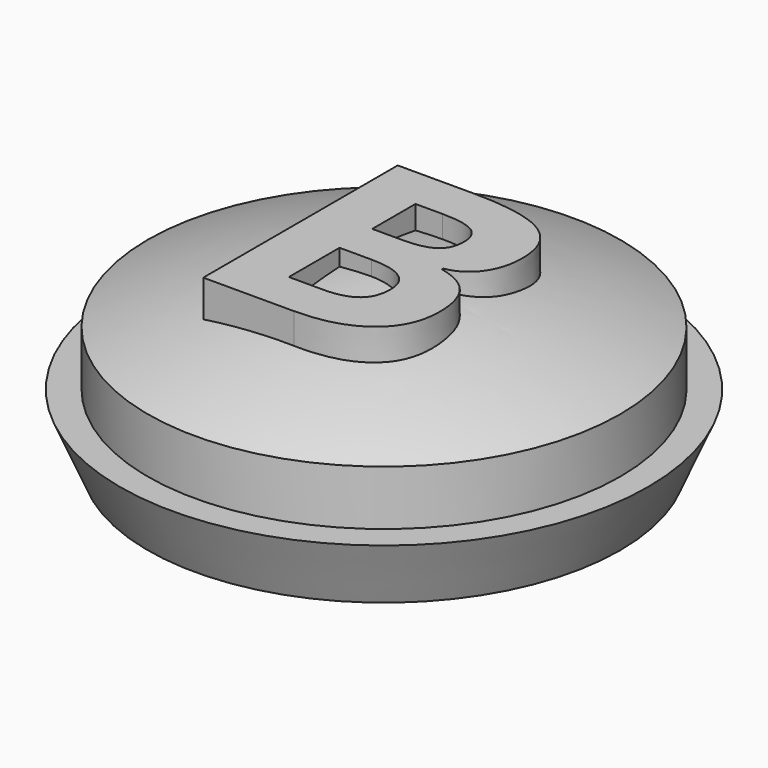
from build123d import *

# Parameters (mm, degrees)
F2_TEXT_SIZE = 15.4926060026
F3_DEPTH     = 3


# Not quite as in the source:
# - Text() gives the source's letters only with a copy of the font that has no kerning and outlines rounded to 1/6400 em; it was checked with that copy


with BuildPart() as f1:
    # F0 (on Front) → F1 (revolve)
    with BuildSketch(Plane.XZ):
        with BuildLine():
            Line((0, 2.3670026567), (0, 0))
            Line((0, 0), (10.75, 0))
            ThreePointArc((10.75, 0), (5.4727971118, 1.6276575482), (0, 2.3670026567))
        make_face()
        Polygon((10.75, 0), (0, 0), (0, -1.2683299238), (9.8515987991, -1.2683299238), (9.8515987991, -5.45), (10.75, -5.45), (12.0183313273, -2.5), (10.75, -2.5), align=None)
    revolve(axis=Axis((0, 0, 0.5493363665), (0, 0, -1)))

    # F2 (on Top) → F3 (join)
    with BuildSketch(Plane.XY):
        with Locations((-5.1787499688, -5.546811597)):
            Text('B', F2_TEXT_SIZE, font='Open Sans', font_style=FontStyle.BOLD, text_align=(TextAlign.LEFT, TextAlign.BOTTOM))
    extrude(amount=F3_DEPTH)


solid = f1.part
